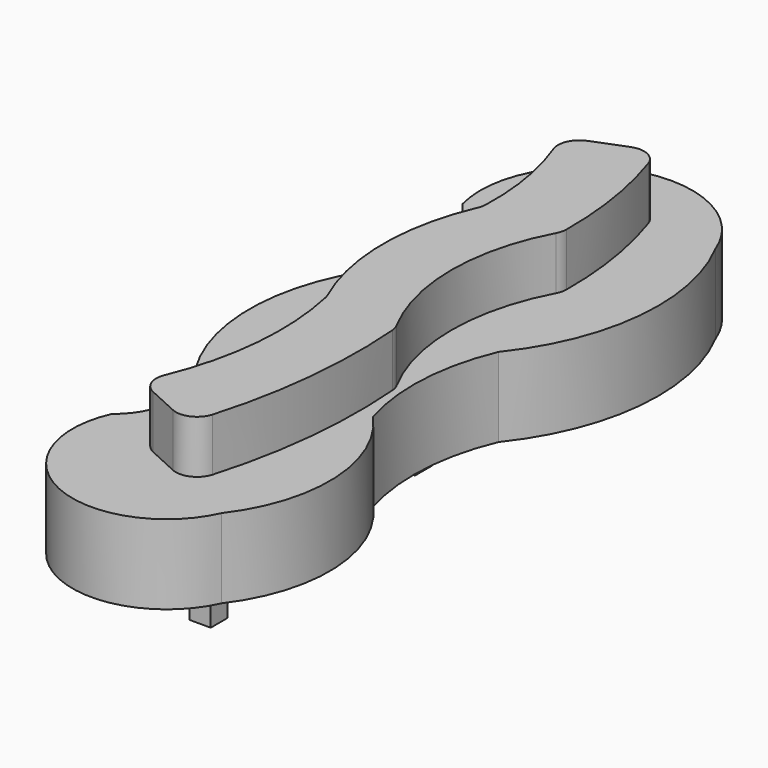
from build123d import *

# Parameters (mm, degrees)
F1_DEPTH = 19.05
F3_DEPTH = 12.7
F4_R     = 5.08
F5_W     = 5.08
F5_H     = 5.08
F6_DEPTH = 7.62


# Not quite as in the source:
# - a feature names something its author has since deleted; it is built from what else it names


with BuildPart() as f1:
    # F0 (on Top) → F1 (new body)
    with BuildSketch(Plane.XY):
        with BuildLine():
            ThreePointArc((-31.6769881083, 69.2702680826), (-41.4338257439, 40.3089202009), (-31.6769881083, 11.3475723192))
            Line((-31.6769881083, 11.3475723192), (3.9428002201, 20.5794945359))
            ThreePointArc((3.9428002201, 20.5794945359), (1.8207183061, 38.3838132659), (5.8883237652, 55.8466762304))
            Line((5.8883237652, 55.8466762304), (-31.6769881083, 69.2702680826))
        make_face()
        with BuildLine():
            ThreePointArc((-36.8869205419, 98.4383374453), (-30.0684968554, 84.6069006975), (-31.6769881083, 69.2702680826))
            Line((-31.6769881083, 69.2702680826), (5.8883237652, 55.8466762304))
            ThreePointArc((5.8883237652, 55.8466762304), (17.3296867389, 83.976336418), (11.5213459358, 113.7831434608))
            Line((11.5213459358, 113.7831434608), (-36.8869205419, 98.4383374453))
        make_face()
        with BuildLine():
            ThreePointArc((-31.6769881083, 11.3475723192), (-29.3116483225, 0.4750905822), (-34.9744334817, -9.1029340401))
            Line((-34.9744334817, -9.1029340401), (6.2283230945, -27.6920832694))
            ThreePointArc((6.2283230945, -27.6920832694), (13.878530495, -3.1399721265), (3.9428002201, 20.5794945359))
            Line((3.9428002201, 20.5794945359), (-31.6769881083, 11.3475723192))
        make_face()
        with BuildLine():
            Line((6.2283230945, -27.6920832694), (-34.9744334817, -9.1029340401))
            ThreePointArc((-34.9744334817, -9.1029340401), (-23.6676298082, -38.9988869429), (6.2283230945, -27.6920832694))
        make_face()
        with BuildLine():
            ThreePointArc((11.5213459358, 113.7831434608), (-19.9807860054, 129.1337402603), (-36.8869205419, 98.4383374453))
            Line((-36.8869205419, 98.4383374453), (11.5213459358, 113.7831434608))
        make_face()
    extrude(amount=F1_DEPTH)

    # F2 (on face) → F3 (join)
    with BuildSketch(Plane.XY.offset(19.05)):
        with BuildLine():
            ThreePointArc((-18.0934686214, 34.295540303), (-16.8286909738, 9.5468310574), (-23.8906592131, -14.2066292465))
            Line((-23.8906592131, -14.2066292465), (-6.6029457375, -22.1301615238))
            ThreePointArc((-6.6029457375, -22.1301615238), (-0.4607343944, 4.7449741554), (0, 32.3092155159))
            Line((0, 32.3092155159), (-18.0934686214, 34.295540303))
        make_face()
        with BuildLine():
            ThreePointArc((-18.0934686214, 80.9150189161), (-23.162661248, 57.6052796096), (-18.0934686214, 34.295540303))
            Line((-18.0934686214, 34.295540303), (0, 32.3092155159))
            ThreePointArc((0, 32.3092155159), (-6.5501688565, 57.2618860751), (0, 82.2145566344))
            ThreePointArc((0, 82.2145566344), (-1.439849547, 100.9781554163), (-6.6029457375, 119.0747916698))
            Line((-6.6029457375, 119.0747916698), (-24.2383088917, 112.1475473046))
            ThreePointArc((-24.2383088917, 112.1475473046), (-19.2665441206, 96.9049694563), (-18.0934686214, 80.9150189161))
        make_face()
    extrude(amount=F3_DEPTH)

    # F4
    f4_edges = [f1.edges().sort_by_distance(p)[0] for p in [
        (-23.890659, -14.206629, 25.4),
        (-6.602946, -22.130162, 25.4),
        (-6.602946, 119.074792, 25.4),
        (-24.238309, 112.147547, 25.4),
        (0, 82.214557, 25.4),
        (0, 32.309216, 25.4),
        (-18.093469, 80.915019, 25.4),
        (-18.093469, 34.29554, 25.4),
    ]]
    fillet(f4_edges, radius=F4_R)

    # F5 (on Top) → F6 (join)
    with BuildSketch(Plane.XY):
        with Locations((-26.6524679592, -24.0524802357)):
            Rectangle(F5_W, F5_H)
        with Locations((-0.8571739626, -22.7268876201)):
            Rectangle(F5_W, F5_H)
        with Locations((-27.3225028068, -5.8132838458)):
            Rectangle(F5_W, F5_H)
        with Locations((-5.4335221648, -10.0806634873)):
            Rectangle(F5_W, F5_H)
        with Locations((-26.5202838928, 9.5173716545)):
            Rectangle(F5_W, F5_H)
        with Locations((-7.7564124949, 14.4977606833)):
            Rectangle(F5_W, F5_H)
        with Locations((-32.2857946157, 33.5665121675)):
            Rectangle(F5_W, F5_H)
        with Locations((-10.6263644993, 33.2580432296)):
            Rectangle(F5_W, F5_H)
        with Locations((-31.4632356167, 49.4136251509)):
            Rectangle(F5_W, F5_H)
        with Locations((-9.5391534269, 49.3687652051)):
            Rectangle(F5_W, F5_H)
        with Locations((-27.4613853544, 70.2730193734)):
            Rectangle(F5_W, F5_H)
        with Locations((-7.6474579982, 71.8173533678)):
            Rectangle(F5_W, F5_H)
        with Locations((-27.4252351373, 89.291498065)):
            Rectangle(F5_W, F5_H)
        with Locations((-5.7547562756, 94.7942361236)):
            Rectangle(F5_W, F5_H)
        with Locations((-29.7734234482, 104.6168133616)):
            Rectangle(F5_W, F5_H)
        with Locations((-7.6474579982, 106.1389820957)):
            Rectangle(F5_W, F5_H)
    extrude(amount=-F6_DEPTH)


solid = f1.part
